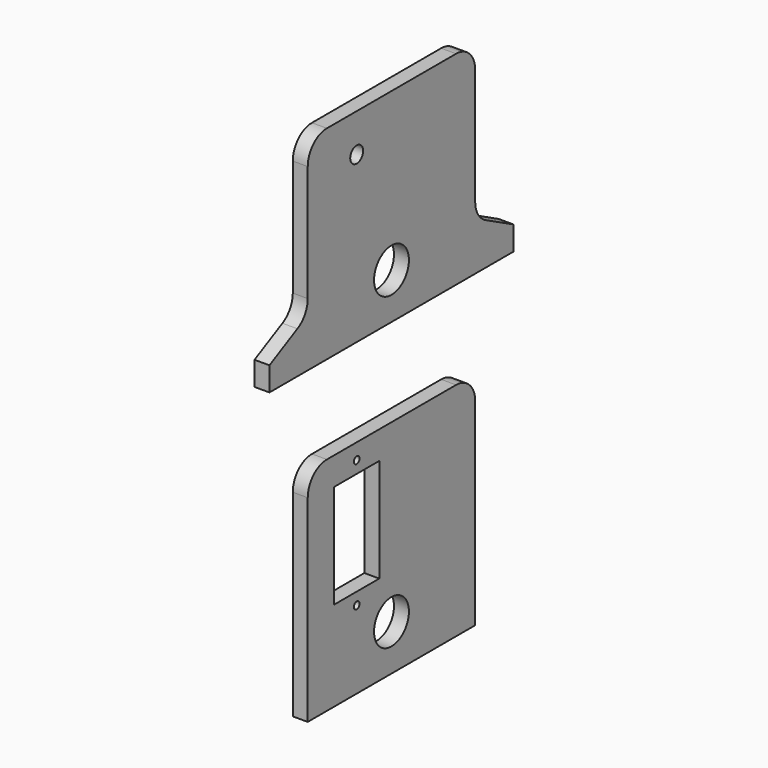
from build123d import *

# Parameters (mm, degrees)
F0_R     = 4.625
F0_R_2   = 1.7145
F1_DEPTH = 3.175
F0_W     = 44.45
F0_H     = 46.99
F0_R_3   = 0.75
F0_W_2   = 12
F0_H_2   = 5.15
F2_R     = 5.08
F2_2_R   = 5.08


# Not quite as in the source:
# - a feature names something its author has since deleted; it is built from what else it names


with BuildPart() as f1:
    # F0 (on Right) → F1 (new body)
    with BuildSketch(Plane.YZ):
        Polygon((-72.304546833, 31.5911603894), (-72.304546833, 21.2748162448), (-27.854546833, 21.2748162448), (-27.854546833, 31.5911603894), (-27.854546833, 64.4548162448), (-59.604546833, 64.4548162448), (-61.3806888302, 64.4548162448), (-72.304546833, 64.4548162448), align=None)
        with Locations((-50.079546833, 30.9798162448)):
            Circle(F0_R, mode=Mode.SUBTRACT)
        with Locations((-59.3140907028, 56.3515170061)):
            Circle(F0_R_2, mode=Mode.SUBTRACT)
        Polygon((-82.464546833, 21.2748162448), (-72.304546833, 21.2748162448), (-72.304546833, 31.5911603894), (-82.464546833, 26.3548162448), align=None)
        Polygon((-27.854546833, 31.5911603894), (-27.854546833, 21.2748162448), (-17.694546833, 21.2748162448), (-17.694546833, 26.3548162448), align=None)
    extrude(amount=F1_DEPTH)

    # F2
    f2_edges = [f1.edges().sort_by_distance(p)[0] for p in [
        (1.5875, -27.854547, 64.454816),
        (1.5875, -72.304547, 64.454816),
        (1.5875, -27.854547, 31.59116),
        (1.5875, -72.304547, 31.59116),
    ]]
    fillet(f2_edges, radius=F2_R)


with BuildPart() as f1b:
    # F0 (on Right) → F1, piece 2 (new body)
    with BuildSketch(Plane.YZ):
        with Locations((-50.079546833, -20.9408289242)):
            Rectangle(F0_W, F0_H)
        Polygon((-53.3140907028, -9.359128163), (-53.3140907028, -25.359128163), (-53.3140907028, -30.509128163), (-65.3140907028, -30.509128163), (-65.3140907028, -25.359128163), (-65.3140907028, -9.359128163), (-65.3140907028, -3.359128163), (-65.3140907028, 1.790871837), (-53.3140907028, 1.790871837), (-53.3140907028, -3.359128163), align=None, mode=Mode.SUBTRACT)
        with Locations((-50.079546833, -34.7308289242)):
            Circle(F0_R, mode=Mode.SUBTRACT)
        Polygon((-59.3140907028, -3.359128163), (-53.3140907028, -3.359128163), (-53.3140907028, 1.790871837), (-65.3140907028, 1.790871837), (-65.3140907028, -3.359128163), align=None)
        with Locations((-59.3140907028, -0.784128163)):
            Circle(F0_R_3, mode=Mode.SUBTRACT)
        with Locations((-59.3140907028, -27.934128163)):
            Rectangle(F0_W_2, F0_H_2)
        with Locations((-59.3140907028, -27.934128163)):
            Circle(F0_R_3, mode=Mode.SUBTRACT)
    extrude(amount=F1_DEPTH)

    # F2#2
    f2_2_edges = [f1b.edges().sort_by_distance(p)[0] for p in [
        (1.5875, -72.304547, 2.554171),
        (1.5875, -27.854547, 2.554171),
    ]]
    fillet(f2_2_edges, radius=F2_2_R)


solid = Compound([f1.part, f1b.part])
